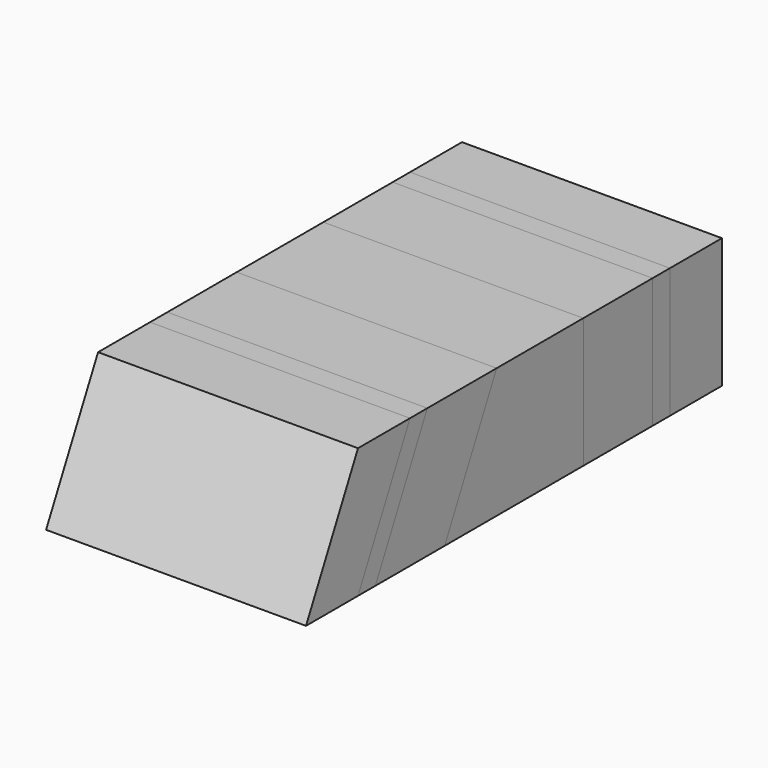
from build123d import *

# Parameters (mm, degrees)
F0_W      = 125
F0_H      = 62.5
F1_DEPTH  = 125
F2_DEPTH  = 62.5
F3_DEPTH  = 93.75
F4_DEPTH  = 31.25
F5_DEPTH  = 83.3333333333
F6_DEPTH  = 41.6666666667
F7_SIZE2  = 31.24999
F7_SIZE   = 62.49999
F8_SIZE2  = 31.24999
F8_SIZE   = 62.49999
F9_SIZE2  = 31.24999
F9_SIZE   = 62.49999
F10_SIZE2 = 31.24999
F10_SIZE  = 62.49999
F11_SIZE2 = 31.24999
F11_SIZE  = 62.49999
F12_SIZE2 = 31.24999
F12_SIZE  = 62.49999


# Not quite as in the source:
# - a fillet or chamfer is up to 0.001 mm smaller than in the source, because OpenCascade refuses the exact size


with BuildPart() as f1:
    # F0 (on Front) → F1 (new body, symmetric)
    with BuildSketch(Plane.XZ):
        Rectangle(F0_W, F0_H)
    extrude(amount=F1_DEPTH, both=True)

    # F7 (size 62.5 and 31.25 in the source; OpenCascade refuses exactly that, so slightly less here)
    f7_edges = [f1.edges().sort_by_distance(p)[0] for p in [
        (0, -125, 31.25),
    ]]
    f7_side = f1.faces().sort_by_distance((0, -125, 0))[0]
    chamfer(f7_edges, length=F7_SIZE, length2=F7_SIZE2, reference=f7_side)


with BuildPart() as f2:
    # F0 (on Front) → F2 (new body, symmetric)
    with BuildSketch(Plane.XZ):
        Rectangle(F0_W, F0_H)
    extrude(amount=F2_DEPTH, both=True)

    # F8 (size 62.5 and 31.25 in the source; OpenCascade refuses exactly that, so slightly less here)
    f8_edges = [f2.edges().sort_by_distance(p)[0] for p in [
        (0, -62.5, 31.25),
    ]]
    f8_side = f2.faces().sort_by_distance((0, -62.5, 0))[0]
    chamfer(f8_edges, length=F8_SIZE, length2=F8_SIZE2, reference=f8_side)


with BuildPart() as f3:
    # F0 (on Front) → F3 (new body, symmetric)
    with BuildSketch(Plane.XZ):
        Rectangle(F0_W, F0_H)
    extrude(amount=F3_DEPTH, both=True)

    # F9 (size 62.5 and 31.25 in the source; OpenCascade refuses exactly that, so slightly less here)
    f9_edges = [f3.edges().sort_by_distance(p)[0] for p in [
        (0, -93.75, 31.25),
    ]]
    f9_side = f3.faces().sort_by_distance((0, -93.75, 0))[0]
    chamfer(f9_edges, length=F9_SIZE, length2=F9_SIZE2, reference=f9_side)


with BuildPart() as f4:
    # F0 (on Front) → F4 (new body, symmetric)
    with BuildSketch(Plane.XZ):
        Rectangle(F0_W, F0_H)
    extrude(amount=F4_DEPTH, both=True)

    # F11 (size 62.5 and 31.25 in the source; OpenCascade refuses exactly that, so slightly less here)
    f11_edges = [f4.edges().sort_by_distance(p)[0] for p in [
        (0, -31.25, 31.25),
    ]]
    f11_side = f4.faces().sort_by_distance((0, -31.25, 0))[0]
    chamfer(f11_edges, length=F11_SIZE, length2=F11_SIZE2, reference=f11_side)


with BuildPart() as f5:
    # F0 (on Front) → F5 (new body, symmetric)
    with BuildSketch(Plane.XZ):
        Rectangle(F0_W, F0_H)
    extrude(amount=F5_DEPTH, both=True)

    # F10 (size 62.5 and 31.25 in the source; OpenCascade refuses exactly that, so slightly less here)
    f10_edges = [f5.edges().sort_by_distance(p)[0] for p in [
        (0, -83.333333, 31.25),
    ]]
    f10_side = f5.faces().sort_by_distance((0, -83.333333, 0))[0]
    chamfer(f10_edges, length=F10_SIZE, length2=F10_SIZE2, reference=f10_side)


with BuildPart() as f6:
    # F0 (on Front) → F6 (new body, symmetric)
    with BuildSketch(Plane.XZ):
        Rectangle(F0_W, F0_H)
    extrude(amount=F6_DEPTH, both=True)

    # F12 (size 62.5 and 31.25 in the source; OpenCascade refuses exactly that, so slightly less here)
    f12_edges = [f6.edges().sort_by_distance(p)[0] for p in [
        (0, -41.666667, 31.25),
    ]]
    f12_side = f6.faces().sort_by_distance((0, -41.666667, 0))[0]
    chamfer(f12_edges, length=F12_SIZE, length2=F12_SIZE2, reference=f12_side)


solid = Compound([f1.part, f2.part, f3.part, f4.part, f5.part, f6.part])
